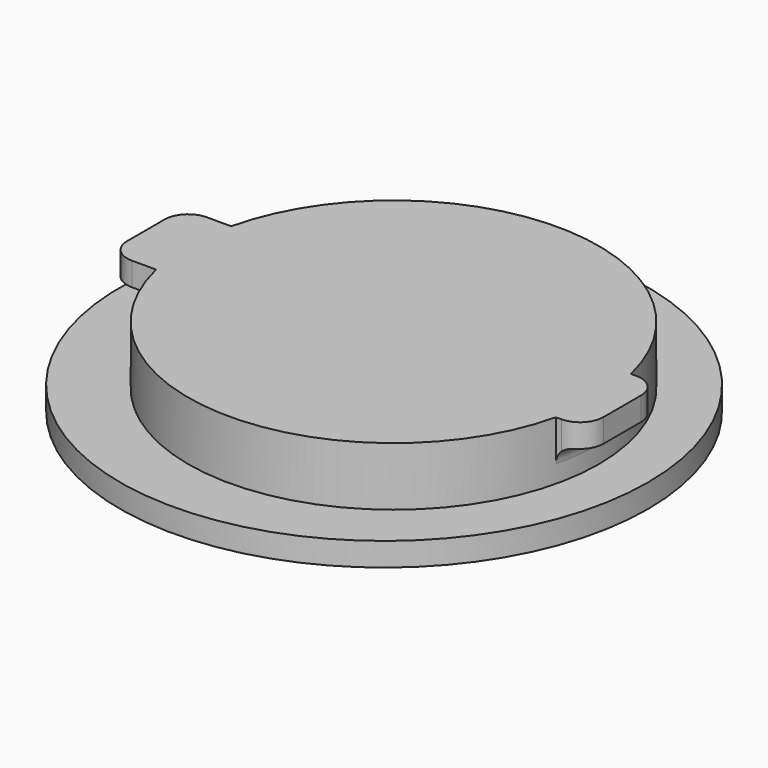
from build123d import *

# Parameters (mm, degrees)
F0_R     = 22.5
F1_DEPTH = 2
F2_R     = 17.5
F3_DEPTH = 5
F5_DEPTH = 2
F6_R     = 1.5
F7_R     = 2
F8_R     = 16
F9_DEPTH = 6
F10_R    = 5.99999


# Not quite as in the source:
# - a fillet or chamfer is up to 0.001 mm smaller than in the source, because OpenCascade refuses the exact size


with BuildPart() as f1:
    # F0 (on Top) → F1 (new body)
    with BuildSketch(Plane.XY):
        Circle(F0_R)
    extrude(amount=F1_DEPTH)

    # F2 (on face) → F3 (join)
    with BuildSketch(Plane.XY.offset(2)):
        with Locations((0.8037949441, 0)):
            Circle(F2_R)
    extrude(amount=F3_DEPTH)

    # F4 (on face) → F5 (join)
    with BuildSketch(Plane.XY.offset(7)):
        with BuildLine():
            Line((-20.3037949441, -4), (-16.2329300933, -4))
            ThreePointArc((-16.2329300933, -4), (-16.6962050559, 0), (-16.2329300933, 4))
            Line((-16.2329300933, 4), (-20.3037949441, 4))
            Line((-20.3037949441, 4), (-20.3037949441, -4))
        make_face()
        with BuildLine():
            Line((-16.2329300933, -4), (17.8405199815, -4))
            ThreePointArc((17.8405199815, -4), (18.1875903893, -2.0133692962), (18.3037949441, 0))
            ThreePointArc((18.3037949441, 0), (18.1875903893, 2.0133692962), (17.8405199815, 4))
            Line((17.8405199815, 4), (-16.2329300933, 4))
            ThreePointArc((-16.2329300933, 4), (-16.6962050559, 0), (-16.2329300933, -4))
        make_face()
        with BuildLine():
            Line((17.8405199815, -4), (20.3037949441, -4))
            Line((20.3037949441, -4), (20.3037949441, 4))
            Line((20.3037949441, 4), (17.8405199815, 4))
            ThreePointArc((17.8405199815, 4), (18.1875903893, 2.0133692962), (18.3037949441, 0))
            ThreePointArc((18.3037949441, 0), (18.1875903893, -2.0133692962), (17.8405199815, -4))
        make_face()
    extrude(amount=-F5_DEPTH)

    # F6
    f6_edges = [f1.edges().sort_by_distance(p)[0] for p in [
        (18.18759, -2.013369, 5),
        (-16.696205, 0, 5),
        (18.18759, 2.013369, 5),
    ]]
    fillet(f6_edges, radius=F6_R)

    # F7
    f7_edges = [f1.edges().sort_by_distance(p)[0] for p in [
        (-20.303795, 4, 6),
        (-20.303795, -4, 6),
        (20.303795, -4, 6),
        (20.303795, 4, 6),
    ]]
    fillet(f7_edges, radius=F7_R)

    # F8 (on face) → F9 (cut)
    with BuildSketch(Plane(origin=(0, 0, 0), x_dir=(1, 0, 0), z_dir=(0, 0, -1))):
        Circle(F8_R)
    extrude(amount=-F9_DEPTH, mode=Mode.SUBTRACT)

    # F10 (radius 6 in the source; OpenCascade refuses exactly that, so slightly less here)
    f10_edges = [f1.edges().sort_by_distance(p)[0] for p in [
        (-16, 0, 6),
    ]]
    fillet(f10_edges, radius=F10_R)

    # F11 (on face) → F12 (join, up to the next surface of F1)
    with BuildSketch(Plane(origin=(0, 0, 0), x_dir=(1, 0, 0), z_dir=(0, 0, -1))):
        with BuildLine():
            Line((15.8034806293, 2.5), (-15.8034806293, 2.5))
            ThreePointArc((-15.8034806293, 2.5), (-16, 0), (-15.8034806293, -2.5))
            Line((-15.8034806293, -2.5), (15.8034806293, -2.5))
            ThreePointArc((15.8034806293, -2.5), (15.9507944954, -1.2538560387), (16, 0))
            ThreePointArc((16, 0), (15.9507944954, 1.2538560387), (15.8034806293, 2.5))
        make_face()
    extrude(until=Until.NEXT, dir=(0, 0, 1))


solid = f1.part
